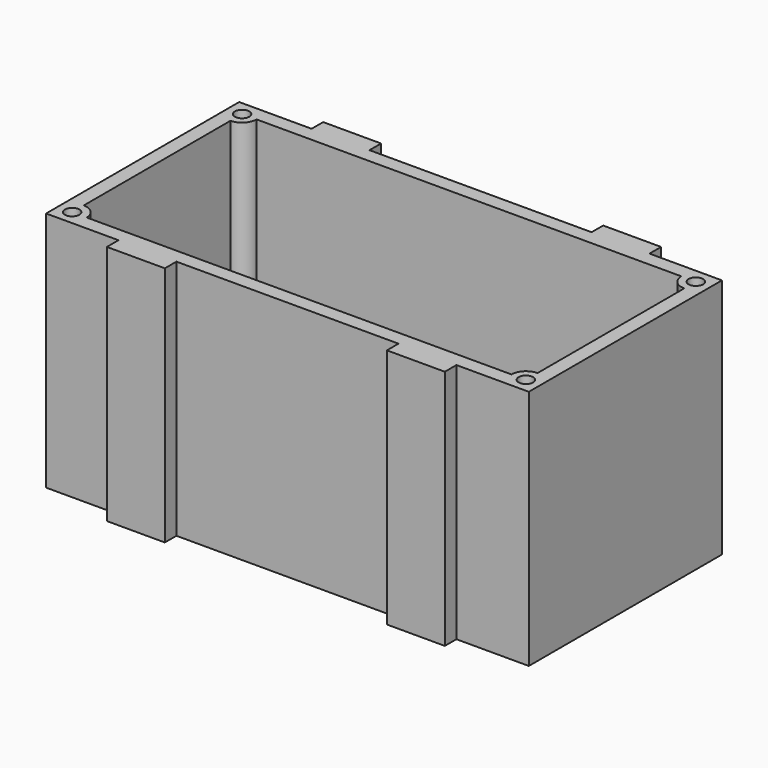
from build123d import *

# Parameters (mm, degrees)
F0_W      = 100
F0_H      = 50
F1_DEPTH  = 5
F2_W      = 100
F2_H      = 50
F3_DEPTH  = 45
F4_W      = 12
F4_H      = 50
F5_DEPTH  = 3
F6_W      = 12
F6_H      = 50
F7_DEPTH  = 3
F8_D      = 3
F8_DEPTH  = 45
F8_TIP    = 0.9012909285
F11_D     = 2
F11_DEPTH = 20
F11_TIP   = 0.600860619


# Not quite as in the source:
# - a feature names something its author has since deleted; it is built from what else it names
# - the program builds the solid bodies; features that only make, move or delete a surface that nothing else refers to are left out


with BuildPart() as f1:
    # F0 (on Top) → F1 (new body)
    with BuildSketch(Plane.XY):
        with Locations((0.7340639085, 12.856667003)):
            Rectangle(F0_W, F0_H)
    extrude(amount=F1_DEPTH)

    # F2 (on face) → F3 (join)
    with BuildSketch(Plane.XY.offset(5)):
        with Locations((0.7340639085, 12.856667003)):
            Rectangle(F2_W, F2_H)
        with BuildLine():
            Line((-46.2659360915, -6.143332997), (-46.2659360915, 31.856667003))
            ThreePointArc((-46.2659360915, 31.856667003), (-44.144615748, 32.7353466595), (-43.2659360915, 34.856667003))
            Line((-43.2659360915, 34.856667003), (44.7340639085, 34.856667003))
            ThreePointArc((44.7340639085, 34.856667003), (45.6127435649, 32.7353466595), (47.7340639085, 31.856667003))
            Line((47.7340639085, 31.856667003), (47.7340639085, -6.143332997))
            ThreePointArc((47.7340639085, -6.143332997), (45.6127435649, -7.0220126534), (44.7340639085, -9.143332997))
            Line((44.7340639085, -9.143332997), (-43.2659360915, -9.143332997))
            ThreePointArc((-43.2659360915, -9.143332997), (-44.144615748, -7.0220126534), (-46.2659360915, -6.143332997))
        make_face(mode=Mode.SUBTRACT)
    extrude(amount=F3_DEPTH)

    # F4 (on face) → F5 (join)
    with BuildSketch(Plane.XZ.offset(12.143332997)):
        with Locations((-28.2659360915, 25)):
            Rectangle(F4_W, F4_H)
        with Locations((29.7340639085, 25)):
            Rectangle(F4_W, F4_H)
    extrude(amount=F5_DEPTH)

    # F6 (on face) → F7 (join)
    with BuildSketch(Plane(origin=(0, 37.856667003, 0), x_dir=(-1, 0, 0), z_dir=(0, 1, 0))):
        with Locations((-29.7340639085, 25)):
            Rectangle(F6_W, F6_H)
        with Locations((28.2659360915, 25)):
            Rectangle(F6_W, F6_H)
    extrude(amount=F7_DEPTH)

    # F8 (one way)
    with BuildSketch(Plane(origin=(0, 0, 5), x_dir=(1, 0, 0), z_dir=(0, 0, -1))):
        with Locations((-46.2659360915, -34.856667003), (-46.2659360915, 9.143332997), (47.7340639085, -34.856667003), (47.7340639085, 9.143332997)):
            Circle(F8_D / 2)
    extrude(amount=-F8_DEPTH, mode=Mode.SUBTRACT)
    with Locations(Plane(origin=(0, 0, 5), x_dir=(1, 0, 0), z_dir=(0, 0, -1))):
        with Locations((-46.2659360915, -34.856667003), (-46.2659360915, 9.143332997), (47.7340639085, -34.856667003), (47.7340639085, 9.143332997)):
            with Locations((0, 0, -(F8_DEPTH + F8_TIP / 2))):  # 118° drill point
                Cone(0, F8_D / 2, F8_TIP, mode=Mode.SUBTRACT)

    # F11
    with Locations(Plane(origin=(0, 0, 0), x_dir=(1, 0, 0), z_dir=(0, 0, -1))):
        with Locations((-42.2659360915, 5.143332997), (43.7340639085, 5.143332997), (43.7340639085, -30.856667003), (-42.2659360915, -30.856667003)):
            Hole(F11_D / 2, depth=F11_DEPTH)
            with Locations((0, 0, -(F11_DEPTH + F11_TIP / 2))):  # 118° drill point
                Cone(0, F11_D / 2, F11_TIP, mode=Mode.SUBTRACT)


solid = f1.part
